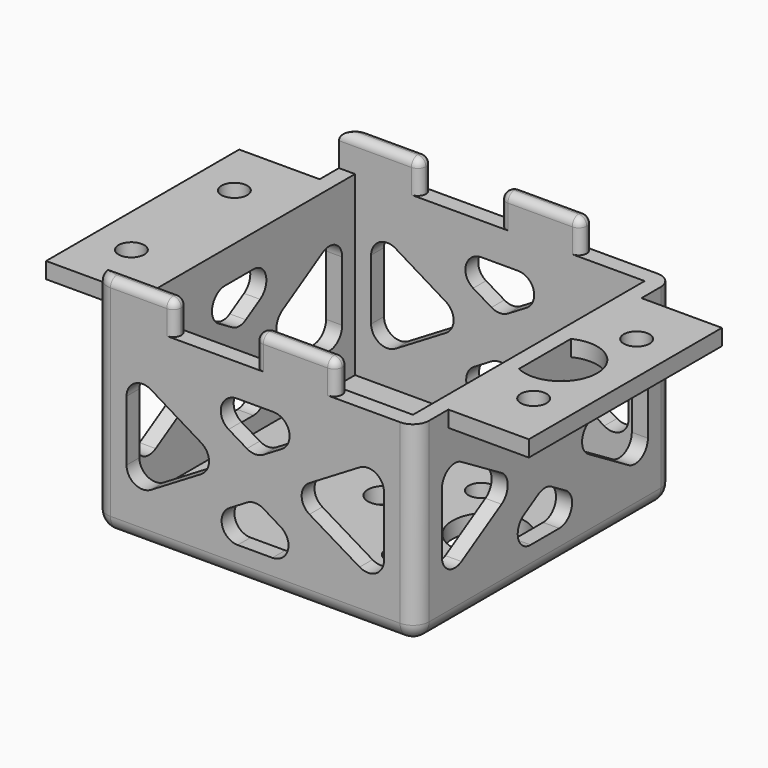
from build123d import *

# Parameters (mm, degrees)
F0_W         = 40
F0_H         = 40
F1_DEPTH     = 2
F2_W         = 40
F2_H         = 40
F2_W_2       = 36
F2_H_2       = 36
F3_DEPTH     = 22
F4_W         = 10
F4_H         = 4
F5_DEPTH     = 2
F6_W         = 10
F6_H         = 4
F7_DEPTH     = 2
F9_DEPTH     = 2
F10_W        = 10
F10_H        = 30
F11_DEPTH    = 2
F12_D        = 3.2
F12_ON_F10_D = 3.2
F13_D        = 3.2
F14_D        = 9
F15_D        = 4
F16_R        = 0.99999
F18_DEPTH    = 40
F20_R        = 2
F21_DEPTH    = 40
F22_R        = 0.99999


# Not quite as in the source:
# - a fillet or chamfer is up to 0.001 mm smaller than in the source, because OpenCascade refuses the exact size


with BuildPart() as f1:
    # F0 (on Top) → F1 (new body)
    with BuildSketch(Plane.XY):
        with Locations((-46.5393099189, 29.7389994189)):
            Rectangle(F0_W, F0_H)
    extrude(amount=F1_DEPTH)

    # F2 (on face) → F3 (join)
    with BuildSketch(Plane.XY.offset(2)):
        with Locations((-46.5393099189, 29.7389994189)):
            Rectangle(F2_W, F2_H)
        with Locations((-46.5393099189, 29.7389994189)):
            Rectangle(F2_W_2, F2_H_2, mode=Mode.SUBTRACT)
    extrude(amount=F3_DEPTH)

    # F4 (on face) → F5 (join, through all)
    with BuildSketch(Plane.XZ.offset(-9.7389994189)):
        with Locations((-41.5393099189, 26)):
            Rectangle(F4_W, F4_H)
        with Locations((-61.5393099189, 26)):
            Rectangle(F4_W, F4_H)
    extrude(amount=-F5_DEPTH)

    # F6 (on face) → F7 (join, through all)
    with BuildSketch(Plane(origin=(0, 49.7389994189, 0), x_dir=(-1, 0, 0), z_dir=(0, 1, 0))):
        with Locations((41.5393099189, 26)):
            Rectangle(F6_W, F6_H)
        with Locations((61.5393099189, 26)):
            Rectangle(F6_W, F6_H)
    extrude(amount=-F7_DEPTH)

    # F8 (on face) → F9 (join)
    with BuildSketch(Plane.XY.offset(24)):
        with BuildLine():
            Line((-16.5393099189, 44.7389994189), (-26.5393099189, 44.7389994189))
            Line((-26.5393099189, 44.7389994189), (-26.5393099189, 33.7701282931))
            ThreePointArc((-26.5393099189, 33.7701282931), (-22.1676016738, 33.5632640541), (-20.0393099189, 29.7389994189))
            ThreePointArc((-20.0393099189, 29.7389994189), (-22.1676016738, 25.9147347837), (-26.5393099189, 25.7078705448))
            Line((-26.5393099189, 25.7078705448), (-26.5393099189, 14.7389994189))
            Line((-26.5393099189, 14.7389994189), (-16.5393099189, 14.7389994189))
            Line((-16.5393099189, 14.7389994189), (-16.5393099189, 44.7389994189))
        make_face()
    extrude(amount=-F9_DEPTH)

    # F10 (on face) → F11 (join)
    with BuildSketch(Plane.XY.offset(24)):
        with Locations((-71.5393099189, 29.7389994189)):
            Rectangle(F10_W, F10_H)
    extrude(amount=-F11_DEPTH)

    # F12 (through all)
    with Locations(Plane.XY.offset(24)):
        with Locations((-21.5393099189, 21.7389994189), (-21.5393099189, 37.7389994189)):
            Hole(F12_D / 2)

    # F12 on F10 (through all)
    with Locations(Plane.XY.offset(24)):
        with Locations((-71.5393099189, 21.7389994189), (-71.5393099189, 37.7389994189)):
            Hole(F12_ON_F10_D / 2)

    # F13 (through all)
    with Locations(Plane(origin=(0, 0, 0), x_dir=(1, 0, 0), z_dir=(0, 0, -1))):
        with Locations((-39.8217954976, -36.4565138402), (-55.3781446837, -38.5778341837), (-53.2568243402, -23.0214849976), (-37.700475154, -20.9001646541)):
            Hole(F13_D / 2)

    # F14 (through all)
    with Locations(Plane(origin=(0, 0, 0), x_dir=(1, 0, 0), z_dir=(0, 0, -1))):
        with Locations((-33.5393099189, -29.7389994189)):
            Hole(F14_D / 2)

    # F15 (through all)
    with Locations(Plane(origin=(0, 0, 0), x_dir=(1, 0, 0), z_dir=(0, 0, -1))):
        with Locations((-46.5393099189, -29.7389994189)):
            Hole(F15_D / 2)

    # F16 (radius 1 in the source; OpenCascade refuses exactly that, so slightly less here)
    f16_edges = [f1.edges().sort_by_distance(p)[0] for p in [
        (-36.53931, 49.738999, 26),
        (-36.53931, 47.738999, 26),
        (-46.53931, 49.738999, 26),
        (-46.53931, 47.738999, 26),
        (-56.53931, 47.738999, 26),
        (-56.53931, 49.738999, 26),
        (-56.53931, 9.738999, 26),
        (-46.53931, 9.738999, 26),
        (-36.53931, 9.738999, 26),
        (-36.53931, 11.738999, 26),
        (-56.53931, 11.738999, 26),
        (-46.53931, 11.738999, 26),
    ]]
    fillet(f16_edges, radius=F16_R)

    # F17 (on face) → F18 (cut, through all)
    with BuildSketch(Plane.YZ.offset(-26.5393099189)):
        with BuildLine():
            Line((16.7679909298, 6.5497756645), (22.9933884033, 10.2850141486))
            ThreePointArc((22.9933884033, 10.2850141486), (23.9643968925, 12), (22.9933884033, 13.7149858514))
            Line((22.9933884033, 13.7149858514), (16.7679909298, 17.4502243355))
            ThreePointArc((16.7679909298, 17.4502243355), (14.7536017889, 17.4756382976), (13.7389994189, 15.7352384841))
            Line((13.7389994189, 15.7352384841), (13.7389994189, 8.2647615159))
            ThreePointArc((13.7389994189, 8.2647615159), (14.7536017889, 6.5243617024), (16.7679909298, 6.5497756645))
        make_face()
        with BuildLine():
            Line((31.9643968925, 20), (27.5136019454, 20))
            ThreePointArc((27.5136019454, 20), (25.586172089, 18.5338671638), (26.4846104345, 16.2850141486))
            Line((26.4846104345, 16.2850141486), (28.7100079081, 14.9497756645))
            ThreePointArc((28.7100079081, 14.9497756645), (29.7389994189, 14.6647615159), (30.7679909298, 14.9497756645))
            Line((30.7679909298, 14.9497756645), (32.9933884033, 16.2850141486))
            ThreePointArc((32.9933884033, 16.2850141486), (33.8918267489, 18.5338671638), (31.9643968925, 20))
        make_face()
        with BuildLine():
            ThreePointArc((45.7389994189, 15.7352384841), (44.7243970489, 17.4756382976), (42.7100079081, 17.4502243355))
            Line((42.7100079081, 17.4502243355), (36.4846104345, 13.7149858514))
            ThreePointArc((36.4846104345, 13.7149858514), (35.5136019454, 12), (36.4846104345, 10.2850141486))
            Line((36.4846104345, 10.2850141486), (42.7100079081, 6.5497756645))
            ThreePointArc((42.7100079081, 6.5497756645), (44.7243970489, 6.5243617024), (45.7389994189, 8.2647615159))
            Line((45.7389994189, 8.2647615159), (45.7389994189, 15.7352384841))
        make_face()
        with BuildLine():
            Line((32.9933884033, 7.7149858514), (30.7679909298, 9.0502243355))
            ThreePointArc((30.7679909298, 9.0502243355), (29.7389994189, 9.3352384841), (28.7100079081, 9.0502243355))
            Line((28.7100079081, 9.0502243355), (26.4846104345, 7.7149858514))
            ThreePointArc((26.4846104345, 7.7149858514), (25.586172089, 5.4661328362), (27.5136019454, 4))
            Line((27.5136019454, 4), (31.9643968925, 4))
            ThreePointArc((31.9643968925, 4), (33.8918267489, 5.4661328362), (32.9933884033, 7.7149858514))
        make_face()
    extrude(amount=-F18_DEPTH, mode=Mode.SUBTRACT)

    # F20
    f20_edges = [f1.edges().sort_by_distance(p)[0] for p in [
        (-26.53931, 49.738999, 12),
        (-66.53931, 49.738999, 14),
        (-46.53931, 49.738999, 0),
        (-26.53931, 29.738999, 0),
        (-66.53931, 29.738999, 0),
        (-46.53931, 9.738999, 0),
        (-66.53931, 9.738999, 14),
        (-26.53931, 9.738999, 12),
    ]]
    fillet(f20_edges, radius=F20_R)

    # F19 (on face) → F21 (cut, through all)
    with BuildSketch(Plane(origin=(0, 49.7389994189, 0), x_dir=(-1, 0, 0), z_dir=(0, 1, 0))):
        with BuildLine():
            ThreePointArc((30.5393099189, 8.2285399911), (31.5539122889, 6.4881401776), (33.5683014297, 6.5135541396))
            Line((33.5683014297, 6.5135541396), (39.80414742, 10.2550617338))
            ThreePointArc((39.80414742, 10.2550617338), (40.7751559092, 11.9700475853), (39.80414742, 13.6850334367))
            Line((39.80414742, 13.6850334367), (33.5683014297, 17.4265410309))
            ThreePointArc((33.5683014297, 17.4265410309), (31.5539122889, 17.4519549929), (30.5393099189, 15.7115551794))
            Line((30.5393099189, 15.7115551794), (30.5393099189, 8.2285399911))
        make_face()
        with BuildLine():
            ThreePointArc((45.5207669248, 14.9198232497), (46.5497584357, 14.6348091011), (47.5787499465, 14.9198232497))
            Line((47.5787499465, 14.9198232497), (49.8540681113, 16.2850141486))
            ThreePointArc((49.8540681113, 16.2850141486), (50.7525064569, 18.5338671638), (48.8250766004, 20))
            Line((48.8250766004, 20), (44.2744402709, 20))
            ThreePointArc((44.2744402709, 20), (42.3470104144, 18.5338671638), (43.24544876, 16.2850141486))
            Line((43.24544876, 16.2850141486), (45.5207669248, 14.9198232497))
        make_face()
        with BuildLine():
            Line((59.5021748451, 17.4931225029), (53.2509853091, 13.7018652759))
            ThreePointArc((53.2509853091, 13.7018652759), (52.288126036, 11.9870366632), (53.259128872, 10.2768060814))
            Line((53.259128872, 10.2768060814), (59.510318408, 6.5260923598))
            ThreePointArc((59.510318408, 6.5260923598), (61.5247075488, 6.5006783977), (62.5393099189, 8.2410782112))
            Line((62.5393099189, 8.2410782112), (62.5393099189, 15.7830491598))
            ThreePointArc((62.5393099189, 15.7830491598), (61.5205667284, 17.5257869697), (59.5021748451, 17.4931225029))
        make_face()
        with BuildLine():
            Line((45.5181768497, 9.0120273198), (43.3714586009, 7.7100733431))
            ThreePointArc((43.3714586009, 7.7100733431), (42.4824386074, 5.4615516209), (44.4085936747, 4))
            Line((44.4085936747, 4), (48.725235218, 4))
            ThreePointArc((48.725235218, 4), (50.6526650744, 5.4661328362), (49.7542267288, 7.7149858514))
            Line((49.7542267288, 7.7149858514), (47.5843034344, 9.0169398281))
            ThreePointArc((47.5843034344, 9.0169398281), (46.5505566539, 9.3019483235), (45.5181768497, 9.0120273198))
        make_face()
    extrude(amount=-F21_DEPTH, mode=Mode.SUBTRACT)

    # F22 (radius 1 in the source; OpenCascade refuses exactly that, so slightly less here)
    f22_edges = [f1.edges().sort_by_distance(p)[0] for p in [
        (-41.53931, 49.738999, 28),
        (-61.039305, 49.738999, 28),
        (-62.039305, 47.738999, 28),
        (-41.53931, 9.738999, 28),
        (-61.039305, 9.738999, 28),
        (-41.53931, 47.738999, 28),
        (-41.53931, 11.738999, 28),
        (-62.039305, 11.738999, 28),
    ]]
    fillet(f22_edges, radius=F22_R)


solid = f1.part
